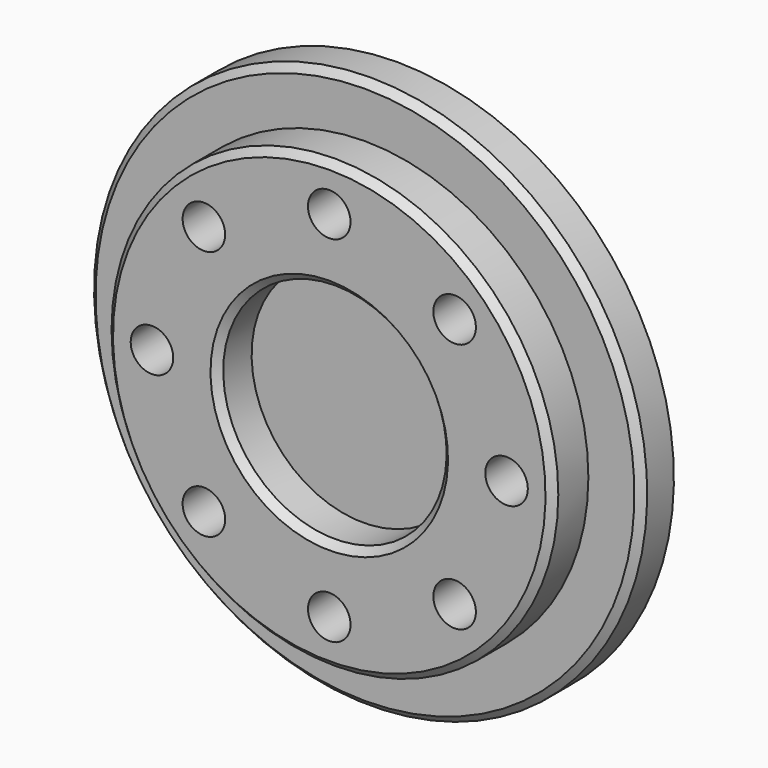
from build123d import *

# Parameters (mm, degrees)
F3_D            = 6
F3_COPIES_COUNT = 8
F4_SIZE         = 1


# Not quite as in the source:
# - a pattern or mirror of a feature is missing from the dataset's text; its kind, count and spacing are read off the source's solid


with BuildPart() as f1:
    # F0 (on Right) → F1 (revolve)
    with BuildSketch(Plane.YZ):
        Polygon((-6, 0), (0, 0), (0, 39), (-5.7, 39), (-5.7, 31.5), (-12, 31.5), (-12, 15.75), (-6, 15.75), align=None)
    revolve(axis=Axis((0, -15.2627385695, 0), (0, -1, 0)))

    # F3 (through all)
    with Locations(Plane(origin=(0, 0, 0), x_dir=(1, 0, 0), z_dir=(0, 1, 0))):
        with Locations((0, -25)):
            f3 = Hole(F3_D / 2)

    # F3_copies: F3 ×8 about axis
    f3_copies_axis = Axis((0, 0, 0), (0, 1, 0))
    for i in range(1, F3_COPIES_COUNT):
        add(f3.rotate(f3_copies_axis, i * 360 / F3_COPIES_COUNT), mode=Mode.SUBTRACT)

    # F4
    f4_edges = [f1.edges().sort_by_distance(p)[0] for p in [
        (0, -12, -15.75),
        (0, -12, -31.5),
        (0, -5.7, -39),
    ]]
    chamfer(f4_edges, length=F4_SIZE)


solid = f1.part
